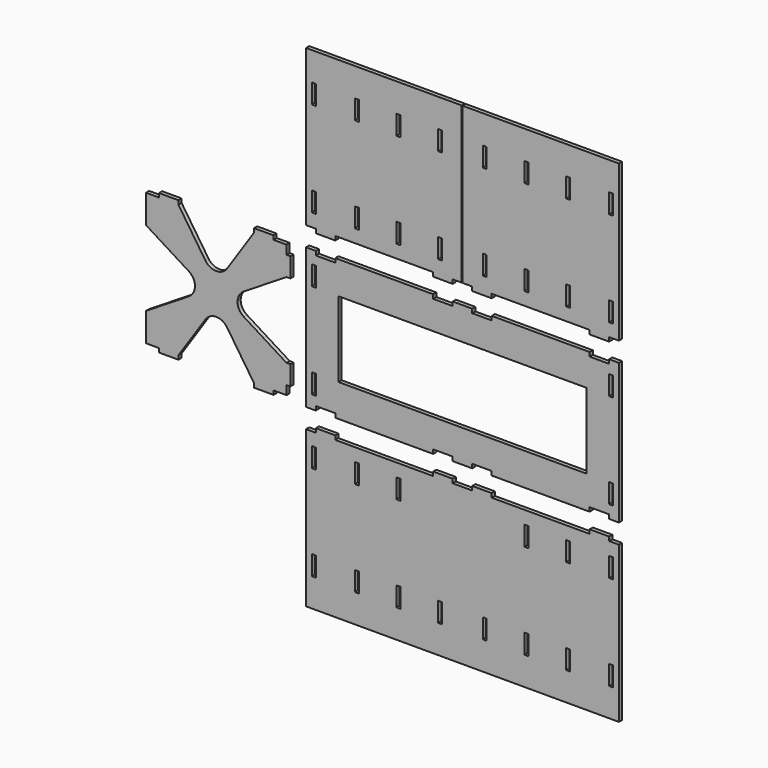
from build123d import *

# Parameters (mm, degrees)
F0_W     = 15.494
F0_H     = 76.2
F0_W_2   = 968.375
F0_H_2   = 295.275
F1_DEPTH = 15.494
F0_W_3   = 76.2
F0_H_3   = 15.748
F0_H_4   = 15.494
F2_R     = 50.8


# Not quite as in the source:
# - a feature names something its author has since deleted; it is built from what else it names


with BuildPart() as f1:
    # F0 (on Front) → F1 (new body)
    with BuildSketch(Plane.XZ):
        Polygon((611.1875, -274.6375), (611.1875, 274.6375), (573.0875, 274.6375), (573.0875, 258.8895), (496.8875, 258.8895), (496.8875, 274.6375), (114.3, 274.6375), (114.3, 258.8895), (38.1, 258.8895), (38.1, 274.6375), (-38.1, 274.6375), (-38.1, 258.8895), (-114.3, 258.8895), (-114.3, 274.6375), (-496.8875, 274.6375), (-496.8875, 258.8895), (-573.0875, 258.8895), (-573.0875, 274.6375), (-611.1875, 274.6375), (-611.1875, -274.6375), (-573.0875, -274.6375), (-573.0875, -258.8895), (-496.8875, -258.8895), (-496.8875, -274.6375), (-114.3, -274.6375), (-114.3, -258.8895), (-38.1, -258.8895), (-38.1, -274.6375), (38.1, -274.6375), (38.1, -258.8895), (114.3, -258.8895), (114.3, -274.6375), (496.8875, -274.6375), (496.8875, -258.8895), (573.0875, -258.8895), (573.0875, -274.6375), align=None)
        with Locations((-580.8345, -185.7375)):
            Rectangle(F0_W, F0_H, mode=Mode.SUBTRACT)
        with Locations((580.8345, -185.7375)):
            Rectangle(F0_W, F0_H, mode=Mode.SUBTRACT)
        with Locations((-580.8345, 185.7375)):
            Rectangle(F0_W, F0_H, mode=Mode.SUBTRACT)
        Rectangle(F0_W_2, F0_H_2, mode=Mode.SUBTRACT)
        with Locations((580.8345, 185.7375)):
            Rectangle(F0_W, F0_H, mode=Mode.SUBTRACT)
    extrude(amount=F1_DEPTH)


with BuildPart() as f1b:
    # F0 (on Front) → F1, piece 2 (new body)
    with BuildSketch(Plane.XZ):
        Polygon((-611.1875, 960.4375), (-611.1875, 350.8375), (-573.0875, 350.8375), (-496.8875, 350.8375), (-114.3, 350.8375), (-38.1, 350.8375), (-3.175, 350.8375), (-3.175, 960.4375), align=None)
        with Locations((-580.8345, 439.7375)):
            Rectangle(F0_W, F0_H, mode=Mode.SUBTRACT)
        with Locations((-412.9405, 439.7375)):
            Rectangle(F0_W, F0_H, mode=Mode.SUBTRACT)
        with Locations((-580.8345, 811.2125)):
            Rectangle(F0_W, F0_H, mode=Mode.SUBTRACT)
        with Locations((-412.9405, 811.2125)):
            Rectangle(F0_W, F0_H, mode=Mode.SUBTRACT)
        with Locations((-250.03125, 439.7375)):
            Rectangle(F0_W, F0_H, mode=Mode.SUBTRACT)
        with Locations((-87.122, 439.7375)):
            Rectangle(F0_W, F0_H, mode=Mode.SUBTRACT)
        with Locations((-250.03125, 811.2125)):
            Rectangle(F0_W, F0_H, mode=Mode.SUBTRACT)
        with Locations((-87.122, 811.2125)):
            Rectangle(F0_W, F0_H, mode=Mode.SUBTRACT)
        with Locations((-534.9875, 342.9635)):
            Rectangle(F0_W_3, F0_H_3)
        with Locations((-76.2, 342.9635)):
            Rectangle(F0_W_3, F0_H_3)
    extrude(amount=F1_DEPTH)


with BuildPart() as f1c:
    # F0 (on Front) → F1, piece 3 (new body)
    with BuildSketch(Plane.XZ):
        Polygon((573.0875, 350.8375), (611.1875, 350.8375), (611.1875, 960.4375), (0, 960.4375), (0, 350.8375), (38.1, 350.8375), (114.3, 350.8375), (496.8875, 350.8375), align=None)
        with Locations((87.122, 439.7375)):
            Rectangle(F0_W, F0_H, mode=Mode.SUBTRACT)
        with Locations((250.03125, 439.7375)):
            Rectangle(F0_W, F0_H, mode=Mode.SUBTRACT)
        with Locations((412.9405, 439.7375)):
            Rectangle(F0_W, F0_H, mode=Mode.SUBTRACT)
        with Locations((580.8345, 439.7375)):
            Rectangle(F0_W, F0_H, mode=Mode.SUBTRACT)
        with Locations((87.122, 811.2125)):
            Rectangle(F0_W, F0_H, mode=Mode.SUBTRACT)
        with Locations((250.03125, 811.2125)):
            Rectangle(F0_W, F0_H, mode=Mode.SUBTRACT)
        with Locations((412.9405, 811.2125)):
            Rectangle(F0_W, F0_H, mode=Mode.SUBTRACT)
        with Locations((580.8345, 811.2125)):
            Rectangle(F0_W, F0_H, mode=Mode.SUBTRACT)
        with Locations((534.9875, 342.9635)):
            Rectangle(F0_W_3, F0_H_3)
        with Locations((76.2, 342.9635)):
            Rectangle(F0_W_3, F0_H_3)
    extrude(amount=F1_DEPTH)


with BuildPart() as f1d:
    # F0 (on Front) → F1, piece 4 (new body)
    with BuildSketch(Plane.XZ):
        Polygon((-687.3875, 223.8375), (-687.3875, 258.8895), (-738.1875, 258.8895), (-814.3875, 258.8895), (-962.025, 38.1), (-1109.6625, 258.8895), (-1185.8625, 258.8895), (-1236.6625, 258.8895), (-1236.6625, 147.6375), (-1000.125, 0), (-1236.6625, -147.6375), (-1236.6625, -258.8895), (-1185.8625, -258.8895), (-1109.6625, -258.8895), (-962.025, -38.1), (-814.3875, -258.8895), (-738.1875, -258.8895), (-687.3875, -258.8895), (-687.3875, -223.8375), (-687.3875, -147.6375), (-923.925, 0), (-687.3875, 147.6375), align=None)
        with Locations((-776.2875, 266.6365)):
            Rectangle(F0_W_3, F0_H_4)
        with Locations((-679.6405, 185.7375)):
            Rectangle(F0_W, F0_H)
        with Locations((-1147.7625, 266.6365)):
            Rectangle(F0_W_3, F0_H_4)
        with Locations((-679.6405, -185.7375)):
            Rectangle(F0_W, F0_H)
        with Locations((-776.2875, -266.6365)):
            Rectangle(F0_W_3, F0_H_4)
        with Locations((-1147.7625, -266.6365)):
            Rectangle(F0_W_3, F0_H_4)
    extrude(amount=F1_DEPTH)

    # F2
    f2_edges = [f1d.edges().sort_by_distance(p)[0] for p in [
        (-1000.125, -7.747, 0),
        (-962.025, -7.747, 38.1),
        (-923.925, -7.747, 0),
        (-962.025, -7.747, -38.1),
    ]]
    fillet(f2_edges, radius=F2_R)


with BuildPart() as f1e:
    # F0 (on Front) → F1, piece 5 (new body)
    with BuildSketch(Plane.XZ):
        with Locations((-76.2, -342.9635)):
            Rectangle(F0_W_3, F0_H_3)
        Polygon((-38.1, -350.8375), (-114.3, -350.8375), (-496.8875, -350.8375), (-573.0875, -350.8375), (-611.1875, -350.8375), (-611.1875, -960.4375), (611.1875, -960.4375), (611.1875, -350.8375), (573.0875, -350.8375), (496.8875, -350.8375), (114.3, -350.8375), (38.1, -350.8375), align=None)
        with Locations((-580.8345, -811.2125)):
            Rectangle(F0_W, F0_H, mode=Mode.SUBTRACT)
        with Locations((-412.9405, -811.2125)):
            Rectangle(F0_W, F0_H, mode=Mode.SUBTRACT)
        with Locations((-580.8345, -439.7375)):
            Rectangle(F0_W, F0_H, mode=Mode.SUBTRACT)
        with Locations((-412.9405, -439.7375)):
            Rectangle(F0_W, F0_H, mode=Mode.SUBTRACT)
        with Locations((-250.03125, -811.2125)):
            Rectangle(F0_W, F0_H, mode=Mode.SUBTRACT)
        with Locations((-87.122, -811.2125)):
            Rectangle(F0_W, F0_H, mode=Mode.SUBTRACT)
        with Locations((87.122, -811.2125)):
            Rectangle(F0_W, F0_H, mode=Mode.SUBTRACT)
        with Locations((250.03125, -811.2125)):
            Rectangle(F0_W, F0_H, mode=Mode.SUBTRACT)
        with Locations((412.9405, -811.2125)):
            Rectangle(F0_W, F0_H, mode=Mode.SUBTRACT)
        with Locations((580.8345, -811.2125)):
            Rectangle(F0_W, F0_H, mode=Mode.SUBTRACT)
        with Locations((-250.03125, -439.7375)):
            Rectangle(F0_W, F0_H, mode=Mode.SUBTRACT)
        with Locations((250.03125, -439.7375)):
            Rectangle(F0_W, F0_H, mode=Mode.SUBTRACT)
        with Locations((412.9405, -439.7375)):
            Rectangle(F0_W, F0_H, mode=Mode.SUBTRACT)
        with Locations((580.8345, -439.7375)):
            Rectangle(F0_W, F0_H, mode=Mode.SUBTRACT)
        with Locations((-534.9875, -342.9635)):
            Rectangle(F0_W_3, F0_H_3)
        with Locations((76.2, -342.9635)):
            Rectangle(F0_W_3, F0_H_3)
        with Locations((534.9875, -342.9635)):
            Rectangle(F0_W_3, F0_H_3)
    extrude(amount=F1_DEPTH)


solid = Compound([f1.part, f1b.part, f1c.part, f1d.part, f1e.part])
